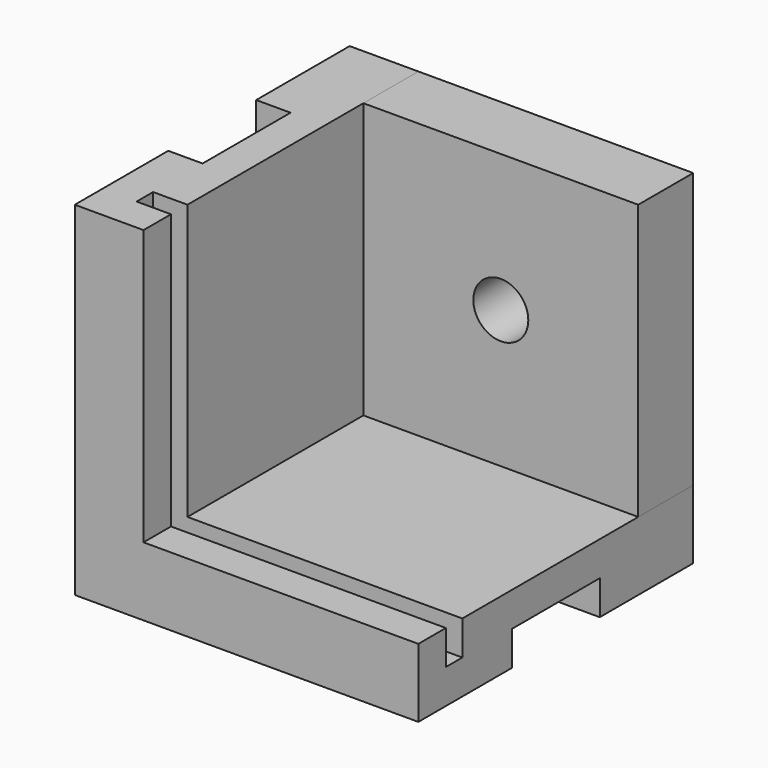
from build123d import *

# Parameters (mm, degrees)
F1_DEPTH  = 50
F2_W      = 3
F2_H      = 40
F3_DEPTH  = 5
F5_DEPTH  = 5
F6_W      = 40
F6_H      = 40
F7_DEPTH  = 10
F8_R      = 4
F9_DEPTH  = 10
F10_W     = 16
F10_H     = 50
F11_DEPTH = 5
F12_W     = 45
F12_H     = 16
F13_DEPTH = 5
F14_R     = 2.5
F15_DEPTH = 25
F16_R     = 2.5
F17_DEPTH = 25


with BuildPart() as f1:
    # F0 (on Front) → F1 (new body)
    with BuildSketch(Plane.XZ):
        Polygon((0, 50), (0, 0), (50, 0), (50, 10), (10, 10), (10, 50), align=None)
    extrude(amount=F1_DEPTH)

    # F2 (on face) → F3 (cut)
    with BuildSketch(Plane.YZ.offset(10)):
        with Locations((-43.5, 30)):
            Rectangle(F2_W, F2_H)
    extrude(amount=-F3_DEPTH, mode=Mode.SUBTRACT)

    # F4 (on face) → F5 (cut)
    with BuildSketch(Plane.XY.offset(10)):
        Polygon((5, -45), (10, -45), (50, -45), (50, -42), (10, -42), (5, -42), align=None)
    extrude(amount=-F5_DEPTH, mode=Mode.SUBTRACT)

    # F10 (on face) → F11 (cut)
    with BuildSketch(Plane(origin=(0, 0, 0), x_dir=(0, -1, 0), z_dir=(-1, 0, 0))):
        with Locations((25, 25)):
            Rectangle(F10_W, F10_H)
    extrude(amount=-F11_DEPTH, mode=Mode.SUBTRACT)

    # F12 (on face) → F13 (cut)
    with BuildSketch(Plane(origin=(0, 0, 0), x_dir=(1, 0, 0), z_dir=(0, 0, -1))):
        with Locations((27.5, 25)):
            Rectangle(F12_W, F12_H)
    extrude(amount=-F13_DEPTH, mode=Mode.SUBTRACT)

    # F14 (on face) → F15 (cut)
    with BuildSketch(Plane(origin=(0, 0, 0), x_dir=(0, -1, 0), z_dir=(-1, 0, 0))):
        with Locations((5, 25)):
            Circle(F14_R)
    extrude(amount=-F15_DEPTH, mode=Mode.SUBTRACT)

    # F16 (on face) → F17 (cut)
    with BuildSketch(Plane(origin=(0, 0, 0), x_dir=(1, 0, 0), z_dir=(0, 0, -1))):
        with Locations((25, 5)):
            Circle(F16_R)
    extrude(amount=-F17_DEPTH, mode=Mode.SUBTRACT)


with BuildPart() as f7:
    # F6 (on face) → F7 (new body)
    with BuildSketch(Plane(origin=(0, 0, 0), x_dir=(-1, 0, 0), z_dir=(0, 1, 0))):
        with Locations((-30, 30)):
            Rectangle(F6_W, F6_H)
    extrude(amount=-F7_DEPTH)

    # F8 (on face) → F9 (cut)
    with BuildSketch(Plane.XZ.offset(10)):
        with Locations((30, 30)):
            Circle(F8_R)
    extrude(amount=-F9_DEPTH, mode=Mode.SUBTRACT)


solid = Compound([f1.part, f7.part])
